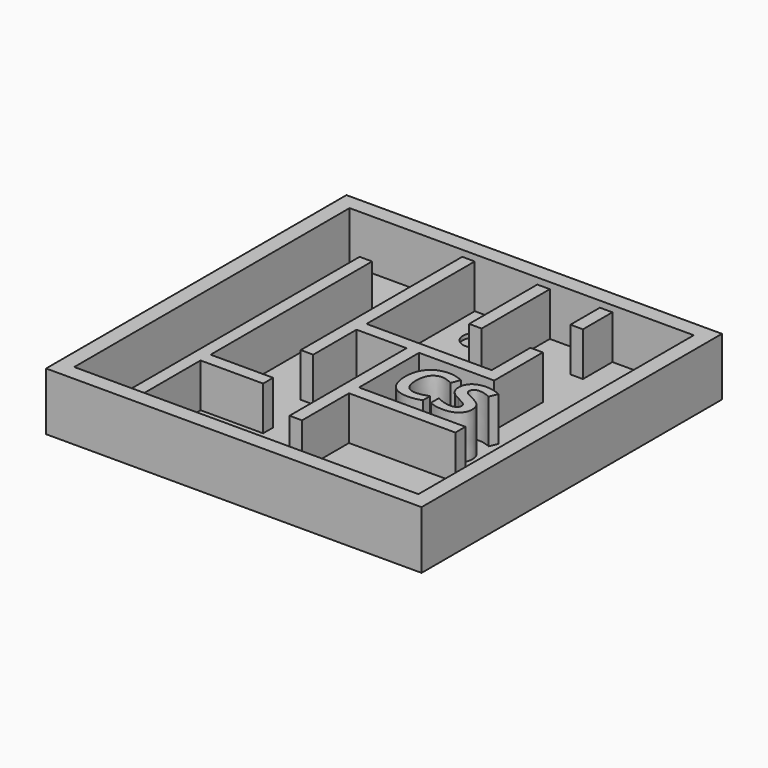
from build123d import *

# Parameters (mm, degrees)
F0_W         = 38.1
F0_H         = 38.1
F1_DEPTH     = 0.79375
F2_W         = 38.1
F2_H         = 38.1
F2_W_2       = 34.925
F2_H_2       = 34.925
F3_DEPTH     = 5.08
F4_W         = 1.27
F4_H         = 8.6465569052
F4_H_2       = 3.7410819112
F5_DEPTH     = 4.445
F6_R         = 1.27
F7_DEPTH     = 0.396875
F8_TEXT_SIZE = 7.0555555556
F9_DEPTH     = 4.445


# Not quite as in the source:
# - Text() gives the source's letters only with a copy of the font that has no kerning and outlines rounded to 1/6400 em; it was checked with that copy


with BuildPart() as f1:
    # F0 (on Top) → F1 (new body)
    with BuildSketch(Plane.XY):
        with Locations((-18.8805037178, 6.3850041287)):
            Rectangle(F0_W, F0_H)
    extrude(amount=F1_DEPTH)

    # F2 (on face) → F3 (join)
    with BuildSketch(Plane.XY.offset(0.79375)):
        with Locations((-18.8805037178, 6.3850041287)):
            Rectangle(F2_W, F2_H)
        with Locations((-18.8805037178, 6.3850041287)):
            Rectangle(F2_W_2, F2_H_2, mode=Mode.SUBTRACT)
    extrude(amount=F3_DEPTH)

    # F4 (on face) → F5 (join)
    with BuildSketch(Plane.XY.offset(0.79375)):
        Polygon((-31.2630037178, 18.7675041287), (-31.2630037178, -11.0774958713), (-29.9930037178, -11.0774958713), (-29.9930037178, -2.9915180057), (-23.6430037178, -2.9915180057), (-23.6430037178, -1.7215180057), (-29.9930037178, -1.7215180057), (-29.9930037178, 18.7675041287), align=None)
        Polygon((-23.6430037178, 23.8475041287), (-24.9130037178, 23.8475041287), (-24.9130037178, 3.3584819943), (-23.6430037178, 3.3584819943), (-23.6430037178, 8.8509472235), (-18.5630037178, 8.8509472235), (-18.5630037178, -5.9974958713), (-17.2930037178, -5.9974958713), (-17.2930037178, -0.0390527765), (-6.4980037178, -0.0390527765), (-6.4980037178, 1.2309472235), (-17.2930037178, 1.2309472235), (-17.2930037178, 8.8509472235), (-9.6730037178, 8.8509472235), (-9.6730037178, 10.1209472235), (-9.6730037178, 15.0264222175), (-10.9430037178, 15.0264222175), (-10.9430037178, 10.1209472235), (-23.6430037178, 10.1209472235), align=None)
        with Locations((-16.6580037178, 19.5242256761)):
            Rectangle(F4_W, F4_H)
        with Locations((-10.3080037178, 21.9769631731)):
            Rectangle(F4_W, F4_H_2)
    extrude(amount=F5_DEPTH)

    # F6 (on face) → F7 (cut)
    with BuildSketch(Plane.XY.offset(0.79375)):
        with Locations((-33.8030037178, -7.2346003726)):
            Circle(F6_R)
        with Locations((-20.4680037178, 19.982073456)):
            Circle(F6_R)
    extrude(amount=-F7_DEPTH, mode=Mode.SUBTRACT)

    # F8 (on face) → F9 (join)
    with BuildSketch(Plane.XY.offset(0.79375)):
        with Locations((-16.0230037178, 2.5009472235)):
            Text('CS', F8_TEXT_SIZE, font='Open Sans', font_style=FontStyle.BOLD, text_align=(TextAlign.LEFT, TextAlign.BOTTOM))
    extrude(amount=F9_DEPTH)


solid = f1.part
